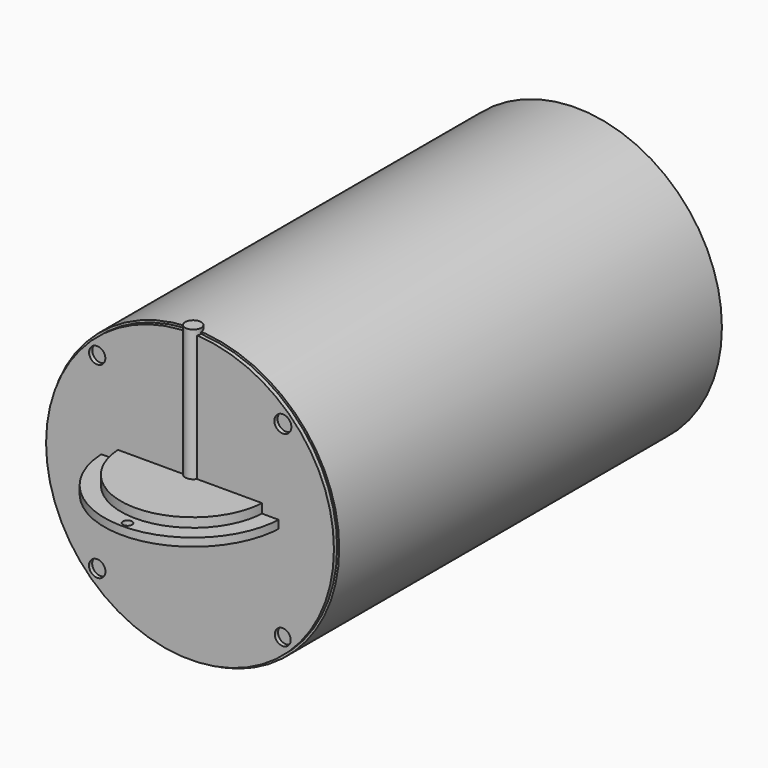
from build123d import *

# Parameters (mm, degrees)
F0_R      = 920.1486376433
F1_DEPTH  = 3014.98
F2_R      = 559.3601435022
F2_R_2    = 28.9882466608
F2_R_3    = 421.8736491985
F3_DEPTH  = 50.8
F4_R      = 455.014896114
F6_DEPTH  = 109.22
F7_R      = 907.1829468917
F7_R_2    = 51.8349054872
F7_R_3    = 50.0342377905
F7_R_4    = 51.2787041201
F7_R_5    = 53.6692639751
F8_DEPTH  = 25.4
F9_R      = 50.0607336969
F10_DEPTH = 939.8


# Not quite as in the source:
# - the program builds the solid bodies; features that only make, move or delete a surface that nothing else refers to are left out


with BuildPart() as f1:
    # F0 (on Front) → F1 (new body)
    with BuildSketch(Plane.XZ):
        Circle(F0_R)
    extrude(amount=-F1_DEPTH)


with BuildPart() as f3:
    # F2 (on Top) → F3 (new body)
    with BuildSketch(Plane.XY):
        Circle(F2_R)
        with Locations((0, -517.4804925919)):
            Circle(F2_R_2, mode=Mode.SUBTRACT)
        Circle(F2_R_3, mode=Mode.SUBTRACT)
        with Locations((0, 515.2065753937)):
            Circle(F2_R_2, mode=Mode.SUBTRACT)
    extrude(amount=F3_DEPTH)


with BuildPart() as f6:
    # F4 (on Top) → F6 (new body)
    with BuildSketch(Plane.XY):
        Circle(F4_R)
    extrude(amount=F6_DEPTH)


with BuildPart() as f8:
    # F7 (on Front) → F8 (new body)
    with BuildSketch(Plane.XZ):
        Circle(F7_R)
        with Locations((-584.9684993263, -591.5097674587)):
            Circle(F7_R_2, mode=Mode.SUBTRACT)
        with Locations((584.4309362264, -592.0409031348)):
            Circle(F7_R_3, mode=Mode.SUBTRACT)
        with Locations((-584.9954457836, 591.4831177773)):
            Circle(F7_R_4, mode=Mode.SUBTRACT)
        with Locations((585.1466364716, 591.3335471873)):
            Circle(F7_R_5, mode=Mode.SUBTRACT)
    extrude(amount=F8_DEPTH)


with BuildPart() as f10:
    # F9 (on Top) → F10 (new body)
    with BuildSketch(Plane.XY):
        Circle(F9_R)
    extrude(amount=F10_DEPTH)


solid = Compound([f1.part, f3.part, f6.part, f8.part, f10.part])
